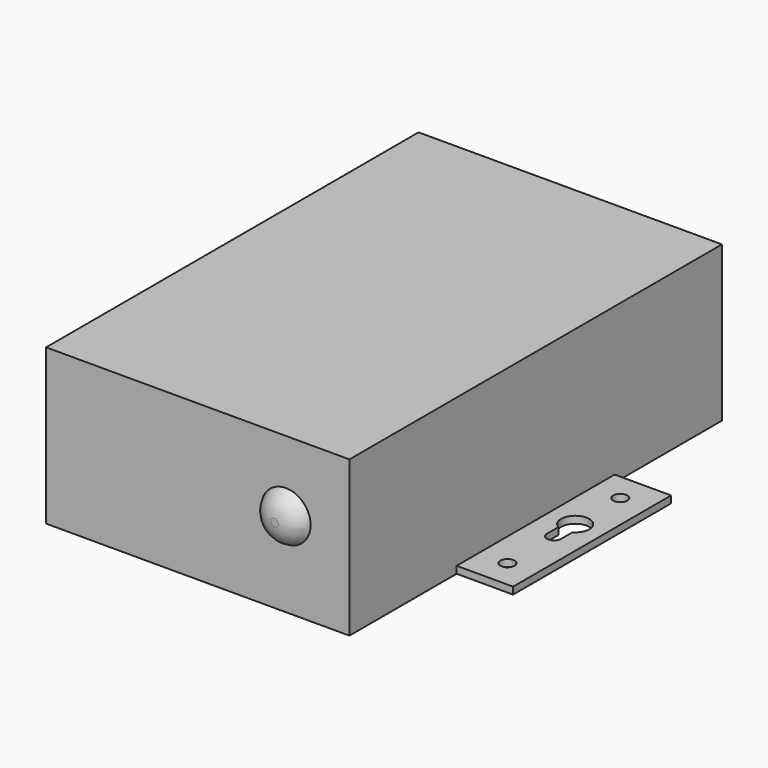
from build123d import *

# Parameters (mm, degrees)
F1_DEPTH = 34.925
F0_W     = 12.7
F0_H     = 44.45
F0_R     = 1.5875
F2_DEPTH = 1.5875
F3_W     = 41.275
F3_H     = 15.875
F4_DEPTH = 11.1125
F5_R     = 5.55625
F6_DEPTH = 3.175


# Not quite as in the source:
# - a fillet or chamfer that OpenCascade refuses, or shapes differently, is made with other operations: its cross-section is extruded or revolved along the edge and cut away or added


with BuildPart() as f1:
    # F0 (on Top) → F1 (new body)
    with BuildSketch(Plane.XY):
        Polygon((34.13125, 22.225), (34.13125, 52.3875), (-34.13125, 52.3875), (-34.13125, 22.225), (-34.13125, -22.225), (-34.13125, -52.3875), (34.13125, -52.3875), (34.13125, -22.225), align=None)
    extrude(amount=F1_DEPTH)

    # F0 (on Top) → F2 (join)
    with BuildSketch(Plane.XY):
        with Locations((-40.48125, 0)):
            Rectangle(F0_W, F0_H)
        with Locations((-40.48125, -15.875)):
            Circle(F0_R, mode=Mode.SUBTRACT)
        with BuildLine():
            Line((-38.89375, 0.425369343), (-38.89375, -2.749630657))
            ThreePointArc((-38.89375, -2.749630657), (-40.48125, -4.337130657), (-42.06875, -2.749630657))
            Line((-42.06875, -2.749630657), (-42.06875, 0.425369343))
            ThreePointArc((-42.06875, 0.425369343), (-40.48125, 6.35), (-38.89375, 0.425369343))
        make_face(mode=Mode.SUBTRACT)
        with Locations((-40.48125, 15.875)):
            Circle(F0_R, mode=Mode.SUBTRACT)
        with Locations((40.48125, 0)):
            Rectangle(F0_W, F0_H)
        with Locations((40.48125, -15.875)):
            Circle(F0_R, mode=Mode.SUBTRACT)
        with BuildLine():
            ThreePointArc((38.89375, 0.425369343), (40.48125, 6.35), (42.06875, 0.425369343))
            Line((42.06875, 0.425369343), (42.06875, -2.749630657))
            ThreePointArc((42.06875, -2.749630657), (40.48125, -4.337130657), (38.89375, -2.749630657))
            Line((38.89375, -2.749630657), (38.89375, 0.425369343))
        make_face(mode=Mode.SUBTRACT)
        with Locations((40.48125, 15.875)):
            Circle(F0_R, mode=Mode.SUBTRACT)
    extrude(amount=F2_DEPTH)

    # F3 (on face) → F4 (join)
    with BuildSketch(Plane(origin=(0, 52.3875, 0), x_dir=(-1, 0, 0), z_dir=(0, 1, 0))):
        with Locations((0, 17.4625)):
            Rectangle(F3_W, F3_H)
    extrude(amount=F4_DEPTH)

    # F5 (on face) → F6 (join)
    with BuildSketch(Plane.XZ.offset(52.3875)):
        with Locations((19.84375, 19.05)):
            Circle(F5_R)
    extrude(amount=F6_DEPTH)

    # F7: fillet of radius 5.08 on 1 edges, made by hand

    # F7_s1 → F7_t2 (revolve, cut)
    with BuildSketch(Plane.XY.offset(19.05)):
        with BuildLine():
            ThreePointArc((25.4, -52.3875), (23.5305202921, -54.6946134838), (20.6907139607, -55.5625))
            Line((20.6907139607, -55.5625), (25.4, -55.5625))
            Line((25.4, -55.5625), (25.4, -52.3875))
        make_face()
    revolve(axis=Axis((19.84375, -55.5625, 19.05), (0, -1, 0)), mode=Mode.SUBTRACT)


solid = f1.part
